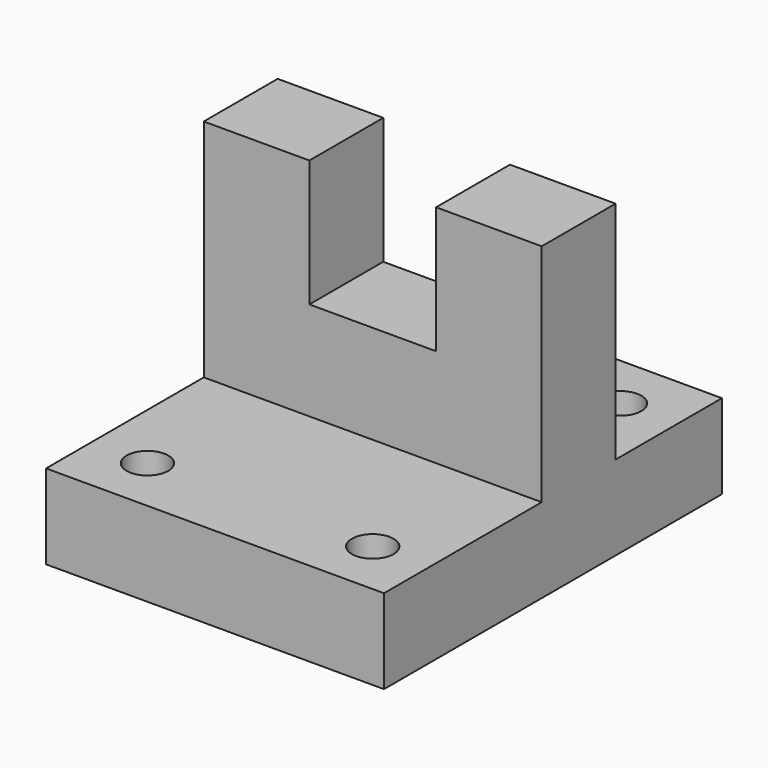
from build123d import *

# Parameters (mm, degrees)
F0_W     = 76.2
F0_H     = 19.05
F1_DEPTH = 20.828
F3_DEPTH = 76.2
F4_R     = 4.699
F5_DEPTH = 41.276


# Not quite as in the source:
# - ends of sketch curves that miss each other by under 0.0002 mm in the source are joined


with BuildPart() as f1:
    # F0 (on Front) → F1 (new body)
    with BuildSketch(Plane.XZ):
        Polygon((-23.8125, 0), (-52.3875009418, 0), (-52.3875009418, 28.575), (-76.2000009418, 28.575), (-76.2000009418, 0), (-76.2, -3.175), (0, -3.175), (0, 0), (0, 28.575), (-23.8125, 28.575), align=None)
        with Locations((-38.1, -12.7)):
            Rectangle(F0_W, F0_H)
    extrude(amount=F1_DEPTH)

    # F2 (on Right) → F3 (join)
    with BuildSketch(Plane.YZ):
        Polygon((0, -22.225), (-20.828, -22.225), (-65.278, -22.225), (-65.278, -41.275), (29.972, -41.275), (29.972, -22.225), align=None)
    extrude(amount=-F3_DEPTH)

    # F4 (on Top) → F5 (cut, through all)
    with BuildSketch(Plane.XY):
        with Locations((-12.7, 17.272)):
            Circle(F4_R)
        with Locations((-12.7, -52.578)):
            Circle(F4_R)
        with Locations((-63.5, -52.578)):
            Circle(F4_R)
        with Locations((-63.5, 17.272)):
            Circle(F4_R)
    extrude(amount=-F5_DEPTH, mode=Mode.SUBTRACT)


solid = f1.part
